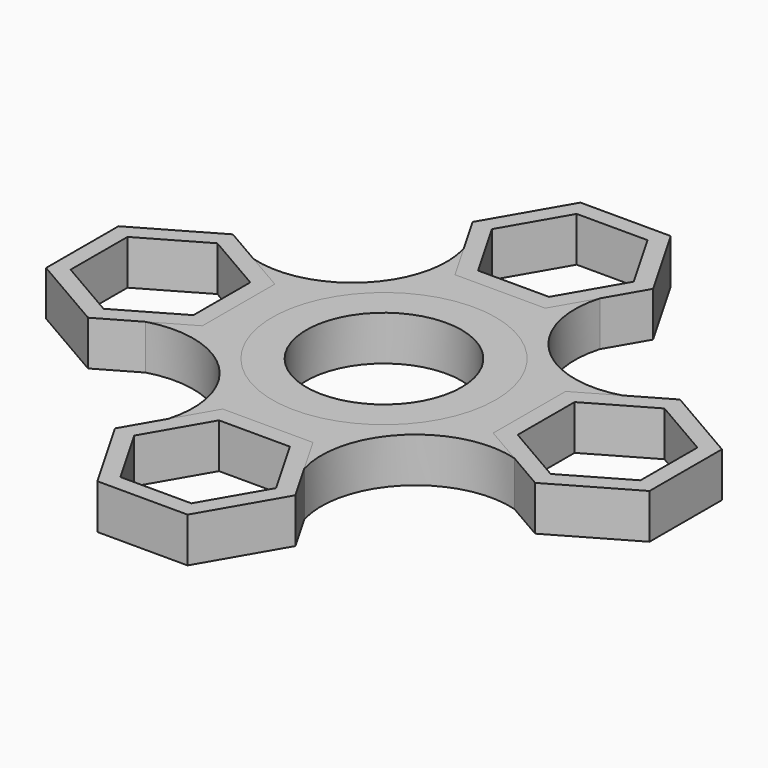
from build123d import *

# Parameters (mm, degrees)
F1_R     = 15.875
F2_DEPTH = 6.35
F0_R     = 15.875
F0_R_2   = 11.0236


# Not quite as in the source:
# - ends of sketch curves that miss each other by under 0.0002 mm in the source are joined


with BuildPart() as f2:
    # F1 (on Top) → F2 (new body)
    with BuildSketch(Plane.XY):
        with BuildLine():
            Line((6.4325482308, -20.6471836189), (9.6068856074, -26.1644869672))
            ThreePointArc((9.6068856074, -26.1644869672), (13.0500837642, -12.9928085244), (26.2491039038, -9.6557918301))
            Line((26.2491039038, -9.6557918301), (26.1792498222, -9.6153210403))
            Line((26.1792498222, -9.6153210403), (20.6278416305, -6.3990469242))
            Line((20.6278416305, -6.3990469242), (20.6375126245, 0.0167504832))
            Line((20.6375126245, 0.0167504832), (20.6471836189, 6.4325482308))
            Line((20.6471836189, 6.4325482308), (26.1644869672, 9.6068856074))
            ThreePointArc((26.1644869672, 9.6068856074), (12.9928085244, 13.0500837642), (9.6557918301, 26.2491039038))
            Line((9.6557918301, 26.2491039038), (9.6153209659, 26.179249694))
            Line((9.6153209659, 26.179249694), (6.3990469242, 20.6278416305))
            Line((6.3990469242, 20.6278416305), (-0.0167505253, 20.6375126245))
            Line((-0.0167505253, 20.6375126245), (-6.4325482308, 20.6471836189))
            Line((-6.4325482308, 20.6471836189), (-9.6068856074, 26.1644869672))
            ThreePointArc((-9.6068856074, 26.1644869672), (-13.0500837642, 12.9928085244), (-26.2491039038, 9.6557918301))
            Line((-26.2491039038, 9.6557918301), (-26.1792498222, 9.6153210403))
            Line((-26.1792498222, 9.6153210403), (-20.6278416305, 6.3990469242))
            Line((-20.6278416305, 6.3990469242), (-20.6374873753, -1.9e-08))
            Line((-20.6374873753, -1.9e-08), (-20.6471836189, -6.4325482308))
            Line((-20.6471836189, -6.4325482308), (-26.1644869672, -9.6068856074))
            ThreePointArc((-26.1644869672, -9.6068856074), (-12.9928085244, -13.0500837642), (-9.6557918301, -26.2491039038))
            Line((-9.6557918301, -26.2491039038), (-9.6153210403, -26.1792498222))
            Line((-9.6153210403, -26.1792498222), (-6.3990469242, -20.6278416305))
            Line((-6.3990469242, -20.6278416305), (0.0167507419, -20.6375126249))
            Line((0.0167507419, -20.6375126249), (6.4325482308, -20.6471836189))
        make_face()
        Circle(F1_R, mode=Mode.SUBTRACT)
    extrude(amount=F2_DEPTH)


with BuildPart() as f2b:
    # F0 (on Top) → F2, piece 2 (new body)
    with BuildSketch(Plane.XY):
        Circle(F0_R)
        Circle(F0_R_2, mode=Mode.SUBTRACT)
    extrude(amount=F2_DEPTH)


with BuildPart() as f2c:
    # F0 (on Top) → F2, piece 3 (new body)
    with BuildSketch(Plane.XY):
        Polygon((6.3990469242, 20.6278416305), (12.831595155, 31.7306580116), (6.4325482308, 42.8528163811), (-6.3990469242, 42.8721583695), (-12.831595155, 31.7693419884), (-6.4325482308, 20.6471836189), align=None)
        Polygon((-5.0278225833, 40.4888387189), (5.0541450385, 40.4736414423), (10.0819676218, 31.7348027234), (5.0278225833, 23.0111612811), (-5.0541450385, 23.0263585577), (-10.0819676218, 31.7651972766), align=None, mode=Mode.SUBTRACT)
    extrude(amount=F2_DEPTH)


with BuildPart() as f2d:
    # F0 (on Top) → F2, piece 4 (new body)
    with BuildSketch(Plane.XY):
        Polygon((31.7693419884, 12.831595155), (20.6471836189, 6.4325482308), (20.6278416305, -6.3990469242), (31.7306580116, -12.831595155), (42.8528163811, -6.4325482308), (42.8721583695, 6.3990469242), align=None)
        Polygon((31.7348027234, -10.0819676218), (23.0111612811, -5.0278225833), (23.0263585577, 5.0541450385), (31.7651972766, 10.0819676218), (40.4888387189, 5.0278225833), (40.4736414423, -5.0541450385), align=None, mode=Mode.SUBTRACT)
    extrude(amount=F2_DEPTH)


with BuildPart() as f2e:
    # F0 (on Top) → F2, piece 5 (new body)
    with BuildSketch(Plane.XY):
        Polygon((12.831595155, -31.7693419884), (6.4325482308, -20.6471836189), (-6.3990469242, -20.6278416305), (-12.831595155, -31.7306580116), (-6.4325482308, -42.8528163811), (6.3990469242, -42.8721583695), align=None)
        Polygon((-10.0819676218, -31.7348027234), (-5.0278225833, -23.0111612811), (5.0541450385, -23.0263585577), (10.0819676218, -31.7651972766), (5.0278225833, -40.4888387189), (-5.0541450385, -40.4736414423), align=None, mode=Mode.SUBTRACT)
    extrude(amount=F2_DEPTH)


with BuildPart() as f2f:
    # F0 (on Top) → F2, piece 6 (new body)
    with BuildSketch(Plane.XY):
        Polygon((-31.7693419884, -12.831595155), (-20.6471836189, -6.4325482308), (-20.6278416305, 6.3990469242), (-31.7306580116, 12.831595155), (-42.8528163811, 6.4325482308), (-42.8721583695, -6.3990469242), align=None)
        Polygon((-31.7348027234, 10.0819676218), (-23.0111612811, 5.0278225833), (-23.0263585577, -5.0541450385), (-31.7651972766, -10.0819676218), (-40.4888387189, -5.0278225833), (-40.4736414423, 5.0541450385), align=None, mode=Mode.SUBTRACT)
    extrude(amount=F2_DEPTH)


solid = Compound([f2.part, f2b.part, f2c.part, f2d.part, f2e.part, f2f.part])
